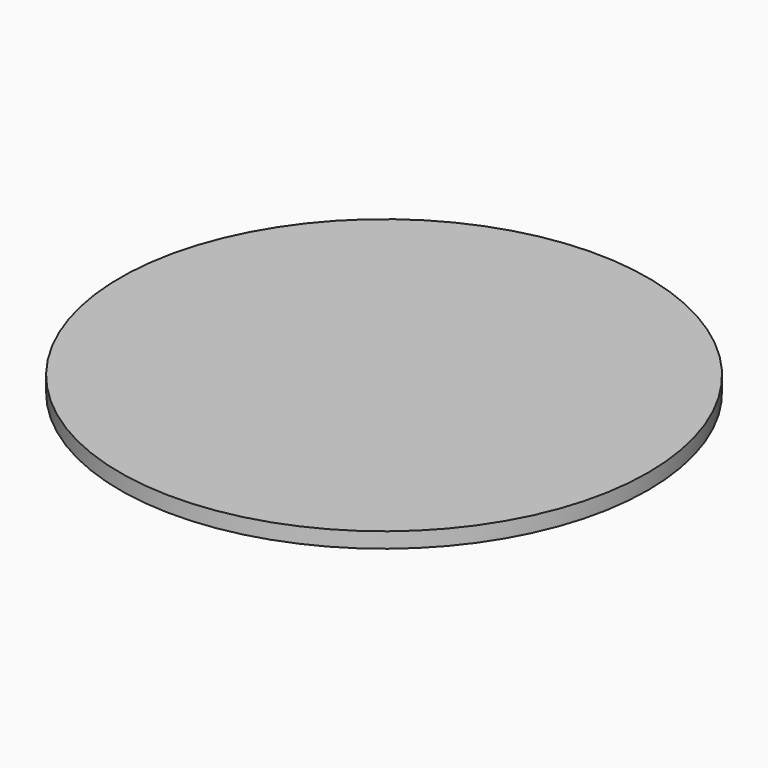
from build123d import *

# Parameters (mm, degrees)
F0_R     = 6
F1_DEPTH = 0.35


# Not quite as in the source:
# - a feature names something its author has since deleted; it is built from what else it names


with BuildPart() as f1:
    # F0 (on Top) → F1 (new body)
    with BuildSketch(Plane.XY):
        Circle(F0_R)
    extrude(amount=-F1_DEPTH)


solid = f1.part
